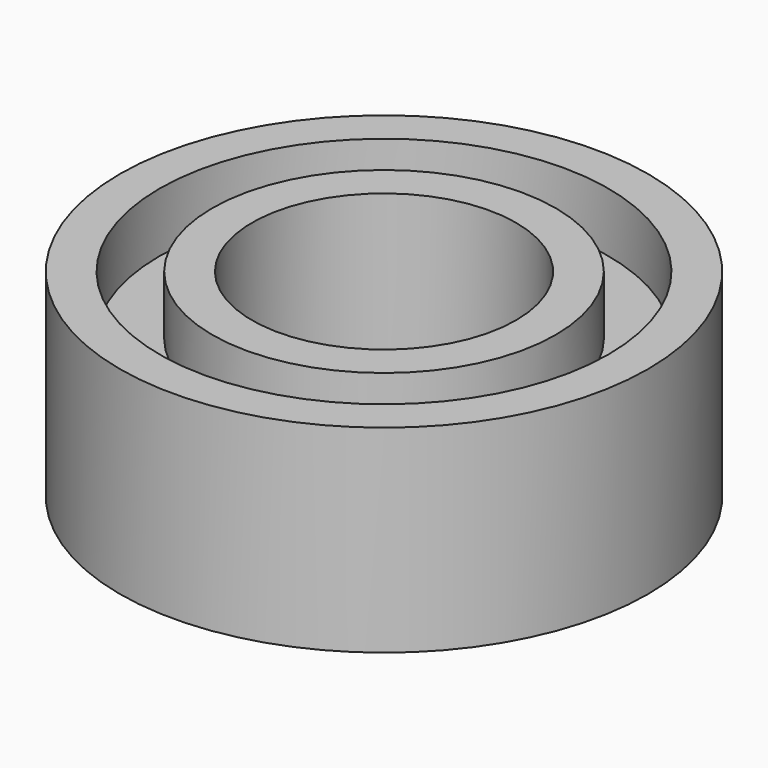
from build123d import *

# Parameters (mm, degrees)
F0_R     = 4
F0_R_2   = 2
F1_DEPTH = 1.5
F2_T     = -0.6
F3_DEPTH = 1.5
F4_T     = 0.6


# Not quite as in the source:
# - a shell that OpenCascade refuses in one call is made with other operations: the cavity is built on its own and cut out


with BuildPart() as f1:
    # F0 (on Top) → F1 (new body)
    with BuildSketch(Plane.XY):
        Circle(F0_R)
        Circle(F0_R_2, mode=Mode.SUBTRACT)
    extrude(amount=F1_DEPTH)

    # F2
    f2_openings = [f1.faces().sort_by_distance(p)[0] for p in [
        (-3.886863, 0, 1.5),
    ]]
    offset(amount=F2_T, openings=f2_openings)

    # F3 (add): a face of the model
    f3_faces = [f1.faces().sort_by_distance(p)[0] for p in [
        (-3.886862915, 0, 0),
    ]]
    extrude(f3_faces, amount=F3_DEPTH)

    # F4: shell of thickness 0.6, made by hand


with BuildPart() as f4_core1:
    # F4_t2: copy of F1
    add(f1.part)

    # the walls: a layer under each face that stays
    f4_faces = [f4_core1.faces().sort_by_distance(p)[0] for p in [
        (-4, 0, 0.75),
        (-4, 0, -0.75),
        (-2.6666666667, -2.6666666667, 1.5),
        (-3.4, 0, 1.05),
        (-2, 0, -0.75),
        (-2.2666666667, -2.2666666667, 0.6),
        (-2, 0, 0.75),
        (-2.6, 0, 1.05),
        (-1.7333333333, -1.7333333333, 1.5),
    ]]
    thicken(f4_faces, amount=-F4_T, mode=Mode.SUBTRACT)

    # F4_s3 → F4_t4 (revolve, cut)
    with BuildSketch(Plane.XZ):
        Polygon((3.394, 0.606), (4, 0.6), (4, 0), (3.4, 0), align=None)
    revolve(axis=Axis((0, 0, 0.6), (0, 0, -1)), mode=Mode.SUBTRACT)

    # F4_s5 → F4_t6 (revolve, cut)
    with BuildSketch(Plane.XZ):
        Polygon((2.606, 0.606), (2.6, 0), (2, 0), (2, 0.6), align=None)
    revolve(axis=Axis((0, 0, 0.6), (0, 0, -1)), mode=Mode.SUBTRACT)


with BuildPart() as f1_1:
    add(f1.part)

    # what is left inside the walls is the cavity
    f4_cavity = [f4_core1.part.solids().sort_by_distance(p)[0] for p in [
        (-3.394, 0, -1),
    ]]
    add(f4_cavity, mode=Mode.SUBTRACT)


solid = f1_1.part
